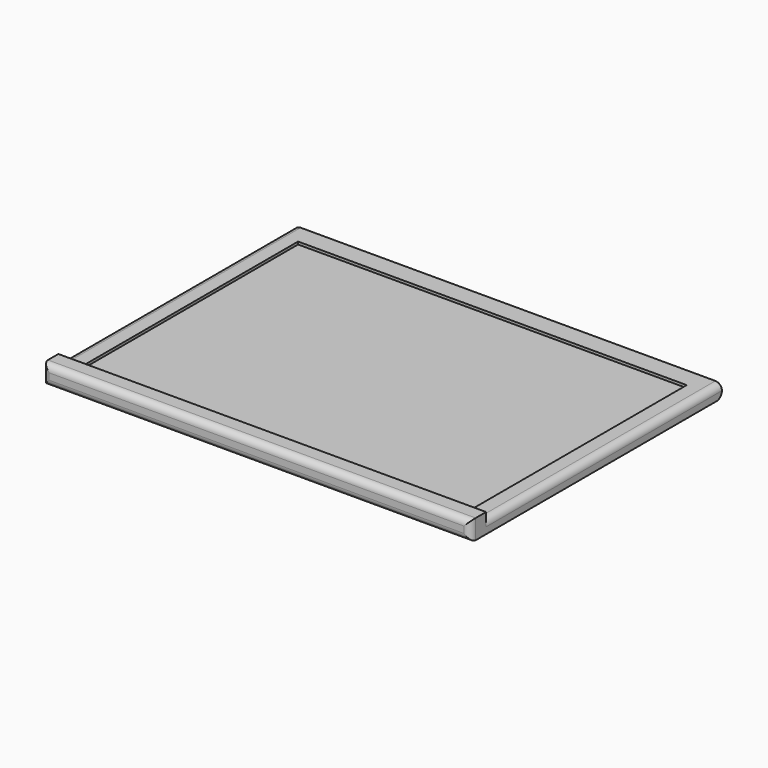
from build123d import *

# Parameters (mm, degrees)
F1_DEPTH = 10
F0_W     = 298
F0_H     = 211
F2_DEPTH = 8
F3_DEPTH = 15
F4_R     = 4.99999


# Not quite as in the source:
# - a fillet or chamfer is up to 0.001 mm smaller than in the source, because OpenCascade refuses the exact size


with BuildPart() as f1:
    # F0 (on Top) → F1 (new body)
    with BuildSketch(Plane.XY):
        Polygon((-149, -105.5), (-149, 105.5), (149, 105.5), (149, -105.5), (164, -105.5), (164, 120.5), (-164, 120.5), (-164, -105.5), align=None)
    extrude(amount=F1_DEPTH)

    # F0 (on Top) → F2 (join)
    with BuildSketch(Plane.XY):
        Rectangle(F0_W, F0_H)
    extrude(amount=F2_DEPTH)

    # F0 (on Top) → F3 (join)
    with BuildSketch(Plane.XY):
        Polygon((149, -105.5), (-149, -105.5), (-164, -105.5), (-164, -120.5), (164, -120.5), (164, -105.5), align=None)
    extrude(amount=F3_DEPTH)

    # F4 (radius 5 in the source; OpenCascade refuses exactly that, so slightly less here)
    f4_edges = [f1.edges().sort_by_distance(p)[0] for p in [
        (0, 120.5, 0),
        (-164, 7.5, 10),
        (164, 7.5, 10),
        (0, -120.5, 15),
        (164, -120.5, 7.5),
        (-164, -120.5, 7.5),
        (0, -120.5, 0),
    ]]
    fillet(f4_edges, radius=F4_R)


solid = f1.part
